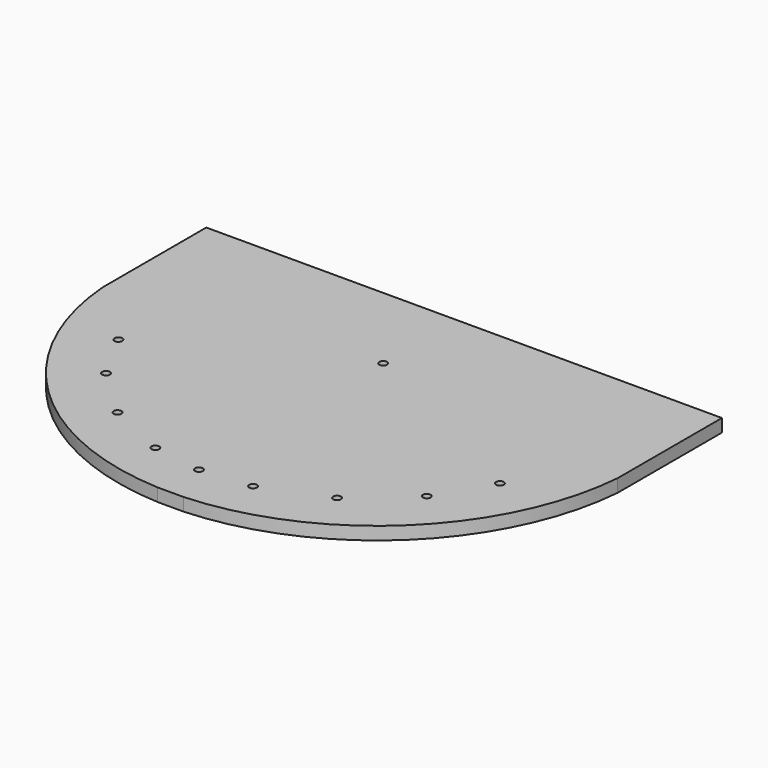
from build123d import *

# Parameters (mm, degrees)
F1_DEPTH = 5
F2_R     = 1.5
F3_DEPTH = 25


# Not quite as in the source:
# - a feature names something its author has since deleted; it is built from what else it names


with BuildPart() as f1:
    # F0 (on Top) → F1 (new body)
    with BuildSketch(Plane.XY):
        with BuildLine():
            ThreePointArc((-97.4828772247, 0), (-67.2370800722, -63.7098067384), (-2.5426874445, -91.7879705417))
            Line((-2.5426874445, -91.7879705417), (7.5769329952, -91.7879705417))
            ThreePointArc((7.5769329952, -91.7879705417), (72.2713256229, -63.7098067384), (102.5171227753, 0))
            Line((102.5171227753, 0), (102.5171227753, 50.5402684212))
            Line((102.5171227753, 50.5402684212), (-97.4828772247, 50.5402684212))
            Line((-97.4828772247, 50.5402684212), (-97.4828772247, 0))
        make_face()
    extrude(amount=F1_DEPTH)

    # F2 (on face) → F3 (cut)
    with BuildSketch(Plane.XY.offset(5)):
        with Locations((-72.3256510152, -23.5000285577)):
            Circle(F2_R)
        with Locations((-61.4798521783, -43.0486559433)):
            Circle(F2_R)
        with Locations((-42.6908970166, -60.9689194803)):
            Circle(F2_R)
        with Locations((-19.2692746164, -71.9139118934)):
            Circle(F2_R)
        with Locations((0, -74.8913536115)):
            Circle(F2_R)
        with Locations((19.5851995713, -73.0929598765)):
            Circle(F2_R)
        with Locations((44.2583380034, -63.2074572013)):
            Circle(F2_R)
        with Locations((64.7310261921, -45.3251524957)):
            Circle(F2_R)
        with Locations((76.7870070898, -24.9496110183)):
            Circle(F2_R)
        with Locations((0, 14.4641017541)):
            Circle(F2_R)
    extrude(amount=-F3_DEPTH, mode=Mode.SUBTRACT)


solid = f1.part
